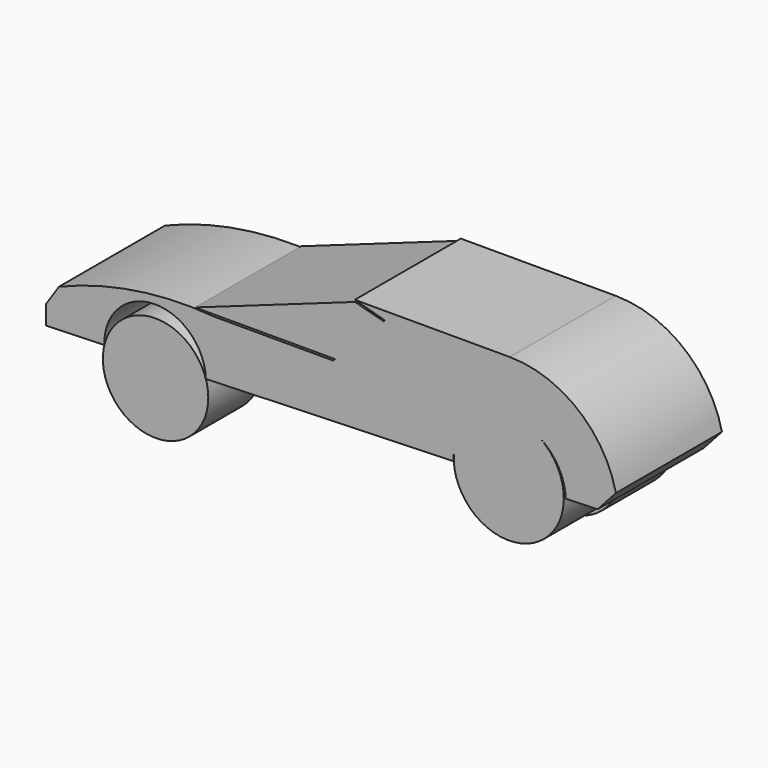
from build123d import *

# Parameters (mm, degrees)
F1_DEPTH     = 12.7
F2_R         = 10.1047698041
F3_DEPTH     = 12.7
F4_R         = 10.5534100151
F5_DEPTH     = 12.7
F6_R         = 10.7401525204
F7_DEPTH     = 12.7
F6_R_2       = 9.7777609661
F9_DEPTH     = 12.7
F10_T1_DEPTH = 39.2535672139


# Not quite as in the source:
# - a fillet or chamfer that OpenCascade refuses, or shapes differently, is made with other operations: its cross-section is extruded or revolved along the edge and cut away or added


with BuildPart() as f1:
    # F0 (on Front) → F1 (new body, symmetric)
    with BuildSketch(Plane.XZ):
        with BuildLine():
            Line((-59.1779053211, 9.7708068788), (-59.1779053211, 3.5027421545))
            Line((-59.1779053211, 3.5027421545), (-48.0088856633, 3.8593999503))
            ThreePointArc((-48.0088856633, 3.8593999503), (-38.5930774629, 13.8963899871), (-28.5560874262, 4.4805817867))
            Line((-28.5560874262, 4.4805817867), (18.9210229876, 5.9966576886))
            ThreePointArc((18.9210229876, 5.9966576886), (29.3376039545, 17.0122475888), (40.4357630105, 6.6836830489))
            Line((40.4357630105, 6.6836830489), (46.5228520607, 6.8780606962))
            Line((46.5228520607, 6.8780606962), (50.0343405137, 10.7586279268))
            ThreePointArc((50.0343405137, 10.7586279268), (42.7319803073, 22.5092393875), (29.6811275184, 27.1001625806))
            Line((29.6811275184, 27.1001625806), (0, 27.1001625806))
            Line((0, 27.1001625806), (5.7562123984, 25.495192036))
            Line((5.7562123984, 25.495192036), (-4.165281076, 15.4858063906))
            Line((-4.165281076, 15.4858063906), (-27.1001625806, 15.4858063906))
            ThreePointArc((-27.1001625806, 15.4858063906), (-43.5123592841, 14.7237458338), (-59.1779053211, 9.7708068788))
        make_face()
    extrude(amount=F1_DEPTH, both=True)

    # F4 (on Front) → F5 (join)
    with BuildSketch(Plane.XZ):
        with Locations((29.4967759401, 6.6367746331)):
            Circle(F4_R)
    extrude(amount=F5_DEPTH)

    # F8 (on Front) → F9 (join, symmetric)
    with BuildSketch(Plane.XZ):
        Polygon((0, 26.7314519733), (-30.6029040366, 15.8545169979), (-3.687096294, 15.8545169979), (5.5306460708, 25.2566132694), align=None)
    extrude(amount=F9_DEPTH, both=True)

    # F10: chamfer of 2.54 on 1 edges, made by hand

    # F10_s2 → F10_t1 (cut)
    with BuildSketch(Plane.XZ.offset(-19.6267836069)):
        with BuildLine():
            Line((-59.2343048388, 7.087548982), (-56.66484646, 10.9375922673))
            Line((-56.66484646, 10.9375922673), (-56.6843383341, 10.9845039593))
            ThreePointArc((-56.6843383341, 10.9845039593), (-57.9365490789, 10.3887043259), (-59.1993652191, 9.8168515612))
            Line((-59.1993652191, 9.8168515612), (-59.2287053211, 9.7708068788))
            ThreePointArc((-59.2287053211, 9.7708068788), (-59.2287053211, 8.4291779304), (-59.2851048388, 7.087548982))
            Line((-59.2851048388, 7.087548982), (-59.2343048388, 7.087548982))
        make_face()
    extrude(amount=F10_T1_DEPTH, mode=Mode.SUBTRACT)


with BuildPart() as f3:
    # F2 (on Front) → F3 (new body)
    with BuildSketch(Plane.XZ):
        with Locations((-38.195622816, 1.4497848184)):
            Circle(F2_R)
    extrude(amount=F3_DEPTH)


with BuildPart() as f7:
    # F6 (on Front) → F7 (new body)
    with BuildSketch(Plane.XZ):
        with Locations((30.234195292, 6.6367746331)):
            Circle(F6_R)
    extrude(amount=-F7_DEPTH)


with BuildPart() as f7b:
    # F6 (on Front) → F7, piece 2 (new body)
    with BuildSketch(Plane.XZ):
        with Locations((-37.9770956933, 1.8435484963)):
            Circle(F6_R_2)
    extrude(amount=-F7_DEPTH)


solid = Compound([f1.part, f3.part, f7.part, f7b.part])
